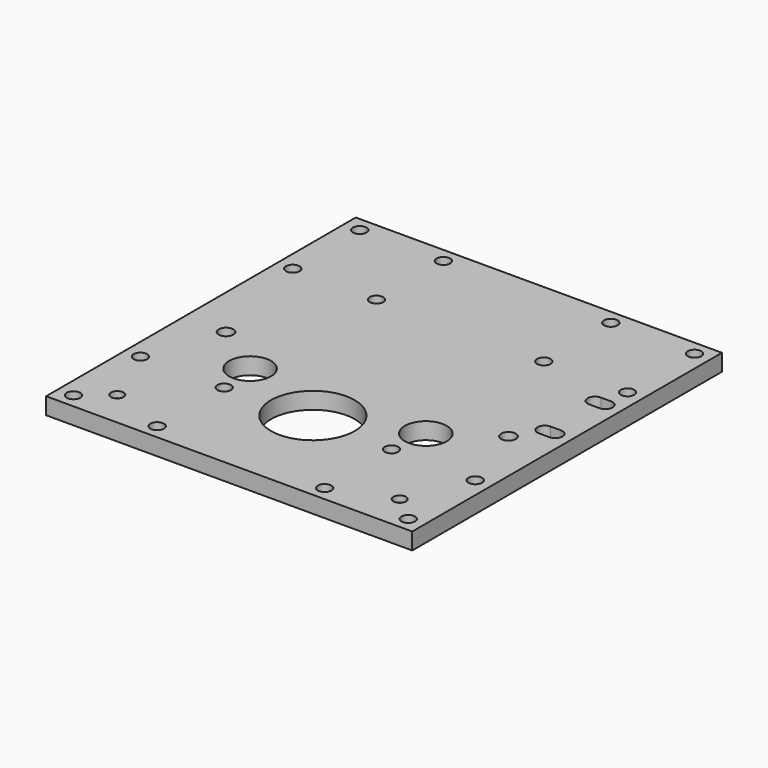
from build123d import *

# Parameters (mm, degrees)
F0_W           = 175
F0_H           = 185
F1_DEPTH       = 8
F2_R           = 3.25
F2_R_2         = 10
F2_R_3         = 3.5
F2_R_4         = 20
F3_DEPTH       = 25
F5_D           = 6
F5_DEPTH       = 15
F5_CBORE_D     = 10
F5_CBORE_DEPTH = 5
F5_TIP         = 1.8025818571


# Not quite as in the source:
# - a feature names something its author has since deleted; it is built from what else it names


with BuildPart() as f1:
    # F0 (on Top) → F1 (new body)
    with BuildSketch(Plane.XY):
        Rectangle(F0_W, F0_H)
    extrude(amount=-F1_DEPTH)

    # F2 (on face) → F3 (cut)
    with BuildSketch(Plane.XY):
        with Locations((-80, 85.5)):
            Circle(F2_R)
        with Locations((-40, 85.5)):
            Circle(F2_R)
        with Locations((-40, 45.5)):
            Circle(F2_R)
        with Locations((-80, 45.5)):
            Circle(F2_R)
        with Locations((40, 85.5)):
            Circle(F2_R)
        with Locations((80, 85.5)):
            Circle(F2_R)
        with Locations((40, 45.5)):
            Circle(F2_R)
        with Locations((80, 45.5)):
            Circle(F2_R)
        with BuildLine():
            Line((77.31, 29), (79.81, 29))
            ThreePointArc((79.81, 29), (83.31, 32.5), (79.81, 36))
            Line((79.81, 36), (74.81, 36))
            ThreePointArc((74.81, 36), (71.31, 32.5), (74.81, 29))
            Line((74.81, 29), (77.31, 29))
        make_face()
        with BuildLine():
            ThreePointArc((79.81, -1), (83.31, 2.5), (79.81, 6))
            Line((79.81, 6), (74.81, 6))
            ThreePointArc((74.81, 6), (71.31, 2.5), (74.81, -1))
            Line((74.81, -1), (79.81, -1))
        make_face()
        with Locations((42, -27.5)):
            Circle(F2_R_2)
        with Locations((40, -45.5)):
            Circle(F2_R)
        with Locations((80, -85.5)):
            Circle(F2_R)
        with Locations((80, -45.5)):
            Circle(F2_R)
        with Locations((40, -85.5)):
            Circle(F2_R)
        with Locations((-40, -85.5)):
            Circle(F2_R)
        with Locations((-80, -85.5)):
            Circle(F2_R)
        with Locations((-80, -45.5)):
            Circle(F2_R)
        with Locations((-40, -45.5)):
            Circle(F2_R)
        with Locations((-42, -27.5)):
            Circle(F2_R_2)
        with Locations((-67.5, -10)):
            Circle(F2_R_3)
        with Locations((0, -42.5)):
            Circle(F2_R_4)
        with Locations((67.5, -10)):
            Circle(F2_R_3)
    extrude(amount=-F3_DEPTH, mode=Mode.SUBTRACT)

    # F5
    with Locations(Plane(origin=(0, 0, -8), x_dir=(1, 0, 0), z_dir=(0, 0, -1))):
        with Locations((-67.5, 75), (67.5, 75)):
            CounterBoreHole(F5_D / 2, F5_CBORE_D / 2, F5_CBORE_DEPTH, depth=F5_DEPTH)
            with Locations((0, 0, -(F5_DEPTH + F5_TIP / 2))):  # 118° drill point
                Cone(0, F5_D / 2, F5_TIP, mode=Mode.SUBTRACT)


solid = f1.part
